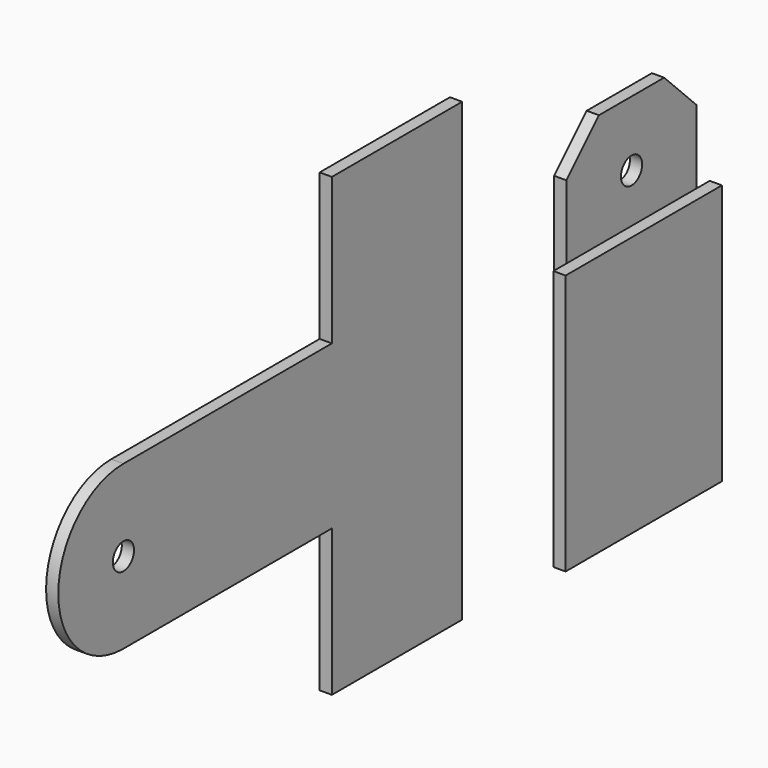
from build123d import *

# Parameters (mm, degrees)
F1_DEPTH = 9.525
F2_SIZE  = 31.75
F3_D     = 20.6375
F4_W     = 12.7
F4_H     = 203.2
F4_W_2   = 63.5
F5_DEPTH = 9.525
F7_DEPTH = 9.525
F8_D     = 20.6375


with BuildPart() as f1:
    # F0 (on Right) → F1 (new body)
    with BuildSketch(Plane.YZ):
        Polygon((101.6, 292.1), (101.6, 0), (165.1, 0), (228.6, 0), (228.6, 292.1), align=None)
    extrude(amount=-F1_DEPTH)

    # F2
    f2_edges = [f1.edges().sort_by_distance(p)[0] for p in [
        (-4.7625, 101.6, 292.1),
        (-4.7625, 228.6, 292.1),
    ]]
    chamfer(f2_edges, length=F2_SIZE)

    # F3 (through all)
    with Locations(Plane.YZ):
        with Locations((165.1, 241.3)):
            Hole(F3_D / 2)

    # F4 (on face) → F5 (join)
    with BuildSketch(Plane.YZ):
        with Locations((95.25, 101.6)):
            Rectangle(F4_W, F4_H)
        with Locations((133.35, 101.6)):
            Rectangle(F4_W_2, F4_H)
        with Locations((196.85, 101.6)):
            Rectangle(F4_W_2, F4_H)
        with Locations((234.95, 101.6)):
            Rectangle(F4_W, F4_H)
    extrude(amount=F5_DEPTH)


with BuildPart() as f7:
    # F6 (on Right) → F7 (new body)
    with BuildSketch(Plane.YZ):
        with BuildLine():
            Line((-127, 0), (0, 0))
            Line((0, 0), (0, 355.6))
            Line((0, 355.6), (-127, 355.6))
            Line((-127, 355.6), (-127, 241.3))
            Line((-127, 241.3), (-330.2, 241.3))
            ThreePointArc((-330.2, 241.3), (-393.7, 177.8), (-330.2, 114.3))
            Line((-330.2, 114.3), (-127, 114.3))
            Line((-127, 114.3), (-127, 0))
        make_face()
    extrude(amount=-F7_DEPTH)

    # F8 (through all)
    with Locations(Plane.YZ):
        with Locations((-330.2, 177.8)):
            Hole(F8_D / 2)


solid = Compound([f1.part, f7.part])
